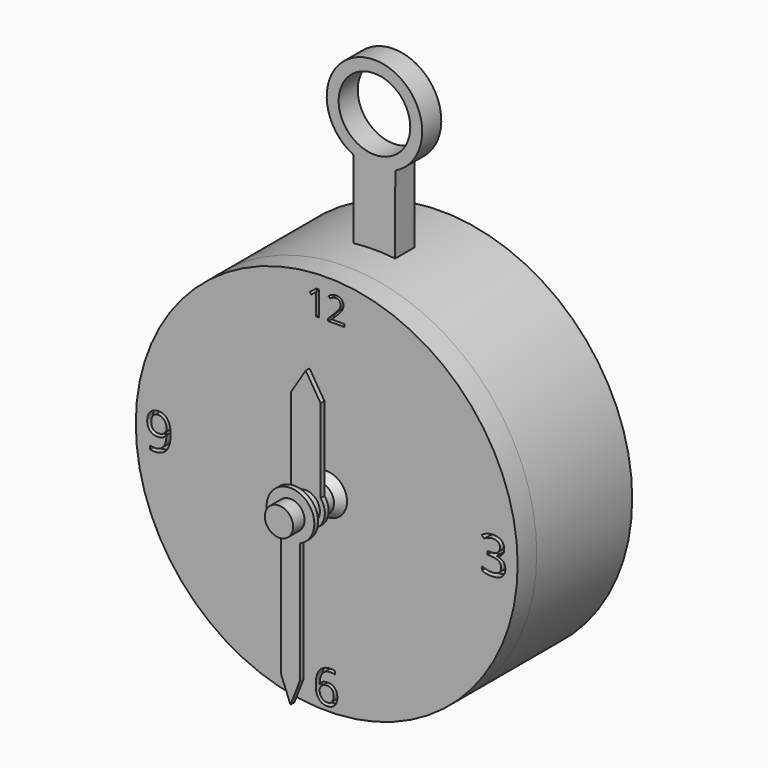
from build123d import *

# Parameters (mm, degrees)
F0_R              = 40
F1_DEPTH          = 12.5
F2_R              = 40
F6_R              = 40
F7_DEPTH          = 5
F8_R              = 4.25
F10_R             = 2.6499999221
F14_D             = 5
F14_DEPTH         = 12
F14_CSINK_D       = 7.5
F14_CSINK_ANGLE   = 120
F14_TIP           = 1.5021515476
F14_2_D           = 5
F14_2_DEPTH       = 12
F14_2_CSINK_D     = 7.5
F14_2_CSINK_ANGLE = 120
F14_2_TIP         = 1.5021515476
F15_R             = 2.9701679383
F16_DEPTH         = 12.5
F18_TEXT_SIZE     = 7.2746955345
F18_TEXT_SIZE_2   = 10.5555555556
F18_TEXT_SIZE_3   = 9.7222222222
F19_DEPTH         = 1.5
F22_DEPTH         = 5
F23_R             = 7.5
F24_DEPTH         = 12.5
F27_DEPTH         = 1
F31_DEPTH         = 1


# Not quite as in the source:
# - Text() gives the source's letters only with a copy of the font that has no kerning and outlines rounded to 1/6400 em; it was checked with that copy


with BuildPart() as f1:
    # F0 (on Front) → F1 (new body, symmetric)
    with BuildSketch(Plane.XZ):
        Circle(F0_R)
    extrude(amount=F1_DEPTH, both=True)

    # F2 (on face) → F5 section 0
    with BuildSketch(Plane(origin=(0, 12.5, 0), x_dir=(-1, 0, 0), z_dir=(0, 1, 0)), mode=Mode.PRIVATE) as f5_s0:
        Circle(F2_R)
    loft([f5_s0.sketch, Vertex(0, 27.5, 0)])

    # F14
    with Locations(Plane.XZ.offset(19.75)):
        with Locations((0, 0)):
            CounterSinkHole(F14_D / 2, F14_CSINK_D / 2, depth=F14_DEPTH, counter_sink_angle=F14_CSINK_ANGLE)
            with Locations((0, 0, -(F14_DEPTH + F14_TIP / 2))):  # 118° drill point
                Cone(0, F14_D / 2, F14_TIP, mode=Mode.SUBTRACT)


with BuildPart() as f7:
    # F6 (on face) → F7 (new body)
    with BuildSketch(Plane.XZ.offset(12.5)):
        Circle(F6_R)
    extrude(amount=F7_DEPTH)

    # F8 (on face) → F11 section 0
    with BuildSketch(Plane.XZ.offset(17.5)):
        Circle(F8_R)
    # F10 (on offset) → F11 section 1
    with BuildSketch(Plane.XZ.offset(19.75)):
        Circle(F10_R)
    loft()

    # F14#2
    with Locations(Plane.XZ.offset(19.75)):
        with Locations((0, 0)):
            CounterSinkHole(F14_2_D / 2, F14_2_CSINK_D / 2, depth=F14_2_DEPTH, counter_sink_angle=F14_2_CSINK_ANGLE)
            with Locations((0, 0, -(F14_2_DEPTH + F14_2_TIP / 2))):  # 118° drill point
                Cone(0, F14_2_D / 2, F14_2_TIP, mode=Mode.SUBTRACT)


with BuildPart() as f16:
    # F15 (on face) → F16 (new body, symmetric)
    with BuildSketch(Plane.XZ.offset(17.5)):
        Circle(F15_R)
    extrude(amount=F16_DEPTH, both=True)

    # F17: cut F7, F1
    add(f7.part, mode=Mode.SUBTRACT)
    add(f1.part, mode=Mode.SUBTRACT)


with BuildPart() as f19:
    # F18 (on face) → F19 (new body)
    with BuildSketch(Plane.XZ.offset(17.5)):
        with Locations((-4.2, 32)):
            Text('12', F18_TEXT_SIZE, font='Open Sans', text_align=(TextAlign.LEFT, TextAlign.BOTTOM))
        with Locations((32, -3.8)):
            Text('3', F18_TEXT_SIZE_2, font='Open Sans', text_align=(TextAlign.LEFT, TextAlign.BOTTOM))
        with Locations((-2.857421875, -39)):
            Text('6', F18_TEXT_SIZE_3, font='Open Sans', text_align=(TextAlign.LEFT, TextAlign.BOTTOM))
        with Locations((-38.1535590278, -3.8)):
            Text('9', F18_TEXT_SIZE_2, font='Open Sans', text_align=(TextAlign.LEFT, TextAlign.BOTTOM))
    extrude(amount=-F19_DEPTH)


with BuildPart() as f7_1:
    add(f7.part)

    # F20: cut F19
    add(f19.part, mode=Mode.SUBTRACT)


with BuildPart() as f1_1:
    add(f1.part)

    # F21 (on Front) → F22 (join)
    with BuildSketch(Plane.XZ):
        with BuildLine():
            Line((4.3411135987, 30), (4.3588864013, 55.9999939255))
            ThreePointArc((4.3588864013, 55.9999939255), (0, 75), (-4.3588864013, 55.9999939255))
            Line((-4.3588864013, 55.9999939255), (-4.3588864013, 30))
            Line((-4.3588864013, 30), (4.3411135987, 30))
        make_face()
    extrude(amount=F22_DEPTH)

    # F23 (on face) → F24 (cut, symmetric)
    with BuildSketch(Plane.XZ.offset(5)):
        with Locations((0, 65)):
            Circle(F23_R)
    extrude(amount=F24_DEPTH, both=True, mode=Mode.SUBTRACT)


with BuildPart() as f27:
    # F26 (on offset) → F27 (new body)
    with BuildSketch(Plane.XZ.offset(22)):
        with BuildLine():
            Line((-3.1224989992, 20), (-3.1224989992, 2.5))
            ThreePointArc((-3.1224989992, 2.5), (0, -4), (3.1224989992, 2.5))
            Line((3.1224989992, 2.5), (3.1224989992, 20))
            Line((3.1224989992, 20), (0, 25))
            Line((0, 25), (-3.1224989992, 20))
        make_face()
    extrude(amount=F27_DEPTH)

    # F28: cut F1
    add(f1_1.part, mode=Mode.SUBTRACT)

    # F33: cut F16
    add(f16.part, mode=Mode.SUBTRACT)


with BuildPart() as f31:
    # F30 (on offset) → F31 (new body)
    with BuildSketch(Plane.XZ.offset(26)):
        with BuildLine():
            Line((1.9595917942, -30), (1.9595917942, -4.6))
            ThreePointArc((1.9595917942, -4.6), (0, 5), (-1.9595917942, -4.6))
            Line((-1.9595917942, -4.6), (-1.9595917942, -30))
            Line((-1.9595917942, -30), (0, -35))
            Line((0, -35), (1.9595917942, -30))
        make_face()
    extrude(amount=F31_DEPTH)

    # F32: cut F1
    add(f1_1.part, mode=Mode.SUBTRACT)

    # F33: cut F16
    add(f16.part, mode=Mode.SUBTRACT)


solid = Compound([f16.part, f7_1.part, f1_1.part, f27.part, f31.part])
